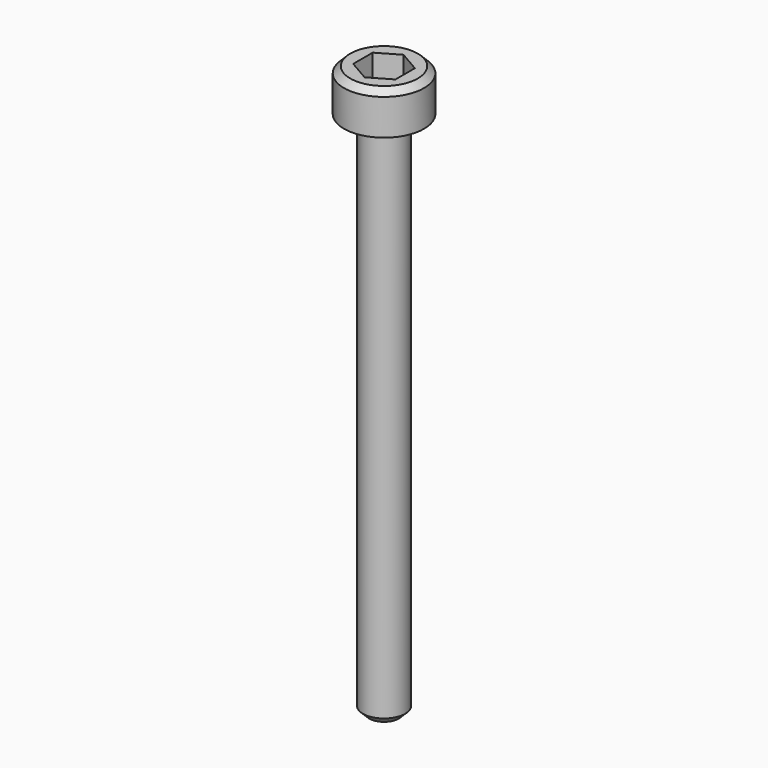
from build123d import *

# Parameters (mm, degrees)
F2_R      = 1
F3_DEPTH  = 25
F2_R_2    = 1.9
F3_FACE_R = 1
F4_DEPTH  = 2
F5_SIZE   = 0.3
F7_DEPTH  = 1.3


with BuildPart() as f3:
    # F2 (on Top) → F3 (new body)
    with BuildSketch(Plane.XY):
        Circle(F2_R)
    extrude(amount=-F3_DEPTH)

    # F2 (on Top) + F3_face (on face) → F4 (join)
    with BuildSketch(Plane.XY):
        Circle(F2_R_2)
        Circle(F2_R, mode=Mode.SUBTRACT)
    with BuildSketch(Plane.XY):
        Circle(F3_FACE_R)
    extrude(amount=F4_DEPTH)

    # F5
    f5_edges = [f3.edges().sort_by_distance(p)[0] for p in [
        (-1, 0, -25),
        (-1.9, 0, 2),
    ]]
    chamfer(f5_edges, length=F5_SIZE)

    # F6 (on face) → F7 (cut)
    with BuildSketch(Plane.XY.offset(2)):
        Polygon((1, -0.5773502692), (1, 0.5773502692), (0, 1.1547005384), (-1, 0.5773502692), (-1, -0.5773502692), (0, -1.1547005384), align=None)
    extrude(amount=-F7_DEPTH, mode=Mode.SUBTRACT)


solid = f3.part
